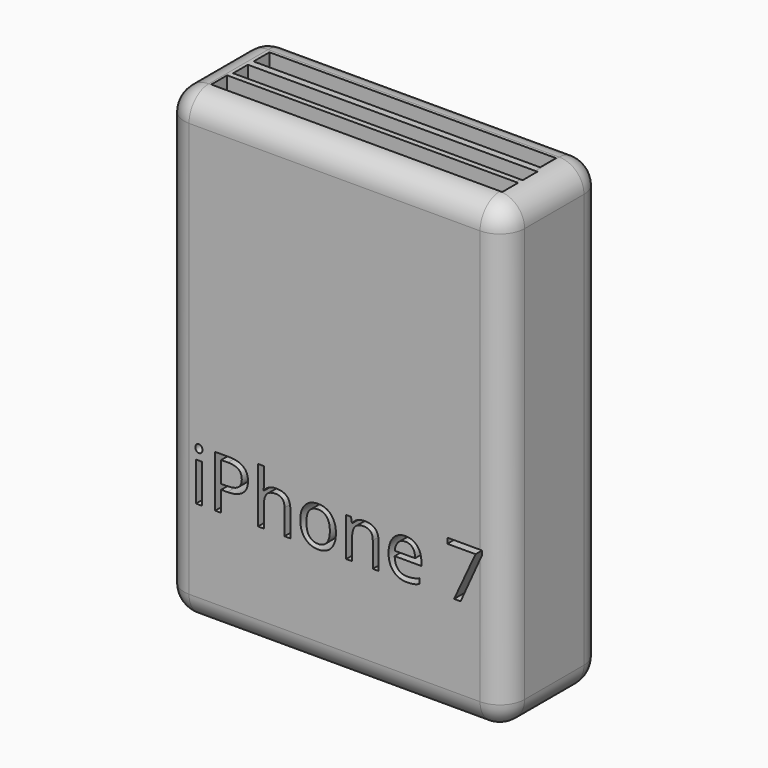
from build123d import *

# Parameters (mm, degrees)
F0_W          = 68.8524655998
F0_H          = 93.8114784658
F1_DEPTH      = 25
F2_R          = 5
F3_R          = 8.880709953
F4_DEPTH      = 4
F5_W          = 57.9508226365
F5_H          = 4.0163928643
F6_DEPTH      = 680.5
F7_W          = 58.5245899856
F7_H          = 3.7295082584
F8_W          = 58.8114783168
F8_H          = 4.0163937956
F9_DEPTH      = 1082.6
F10_TEXT_SIZE = 14.6569994589
F11_DEPTH     = 64.8


# Not quite as in the source:
# - Text() gives the source's letters only with a copy of the font that has no kerning and outlines rounded to 1/6400 em; it was checked with that copy


with BuildPart() as f1:
    # F0 (on Front) → F1 (new body)
    with BuildSketch(Plane.XZ):
        with Locations((0.5737710744, -8.6065586656)):
            Rectangle(F0_W, F0_H)
    extrude(amount=F1_DEPTH)

    # F2
    f2_edges = [f1.edges().sort_by_distance(p)[0] for p in [
        (35.000004, -12.5, 38.299181),
        (0.573771, 0, 38.299181),
        (-33.852462, -12.5, 38.299181),
        (0.573771, -25, 38.299181),
        (-33.852462, 0, -8.606559),
        (35.000004, 0, -8.606559),
        (0.573771, 0, -55.512298),
        (-33.852462, -25, -8.606559),
        (35.000004, -25, -8.606559),
        (0.573771, -25, -55.512298),
        (-33.852462, -12.5, -55.512298),
        (35.000004, -12.5, -55.512298),
    ]]
    fillet(f2_edges, radius=F2_R)

    # F3 (on Front) → F4 (join)
    with BuildSketch(Plane.XZ):
        Circle(F3_R)
    extrude(amount=-F4_DEPTH)

    # F5 (on Top) → F6 (cut)
    with BuildSketch(Plane.XY):
        with Locations((0.8606566116, -7.6024592854)):
            Rectangle(F5_W, F5_H)
    extrude(amount=F6_DEPTH, mode=Mode.SUBTRACT)

    # F7 (on Top) + F8 (on Top) → F9 (cut)
    with BuildSketch(Plane.XY):
        with Locations((1.1475402862, -12.9098366015)):
            Rectangle(F7_W, F7_H)
    with BuildSketch(Plane.XY):
        with Locations((1.0040998459, -17.9303297773)):
            Rectangle(F8_W, F8_H)
    extrude(amount=F9_DEPTH, mode=Mode.SUBTRACT)

    # F10 (on Front) → F11 (cut)
    with BuildSketch(Plane.XZ):
        with Locations((-28.705034405, -33.9211970568)):
            Text('iPhone 7', F10_TEXT_SIZE, font='Open Sans', text_align=(TextAlign.LEFT, TextAlign.BOTTOM))
    extrude(amount=F11_DEPTH, mode=Mode.SUBTRACT)


solid = f1.part
